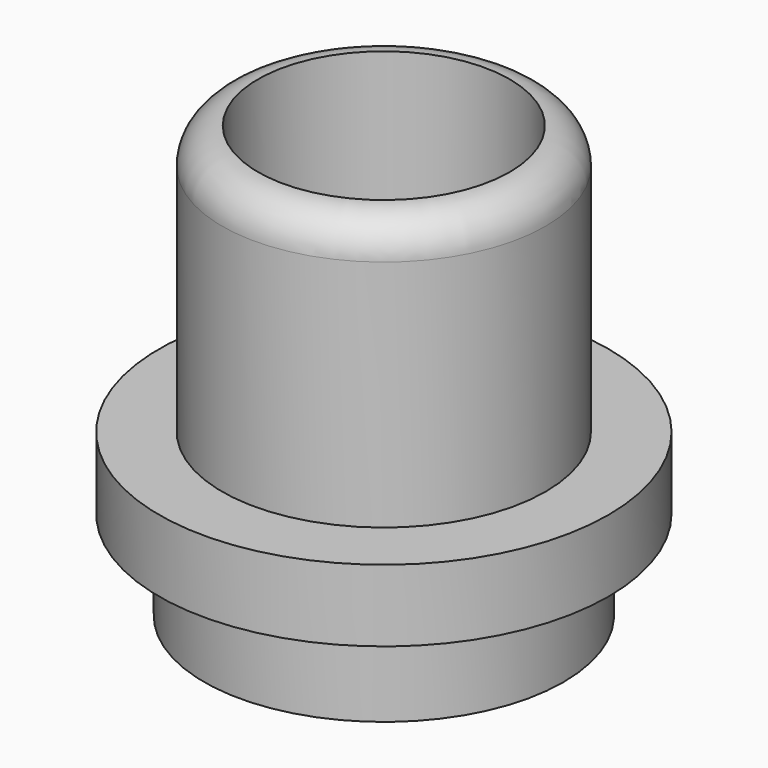
from build123d import *

# Parameters (mm, degrees)
F0_W   = 2
F0_H   = 15
F0_W_2 = 3
F0_H_2 = 5
F2_R   = 1.99999


# Not quite as in the source:
# - a fillet or chamfer is up to 0.001 mm smaller than in the source, because OpenCascade refuses the exact size


with BuildPart() as f1:
    # F0 (on Front) → F1 (revolve)
    with BuildSketch(Plane.XZ):
        with Locations((8, 7.5)):
            Rectangle(F0_W, F0_H)
        Polygon((9, 0), (7, 0), (7, -4), (10, -4), (12.5, -4), (12.5, 0), align=None)
        with Locations((8.5, -6.5)):
            Rectangle(F0_W_2, F0_H_2)
    revolve(axis=Axis((0, 0, 7.5), (0, 0, -1)))

    # F2 (radius 2 in the source; OpenCascade refuses exactly that, so slightly less here)
    f2_edges = [f1.edges().sort_by_distance(p)[0] for p in [
        (-9, 0, 15),
    ]]
    fillet(f2_edges, radius=F2_R)


solid = f1.part
